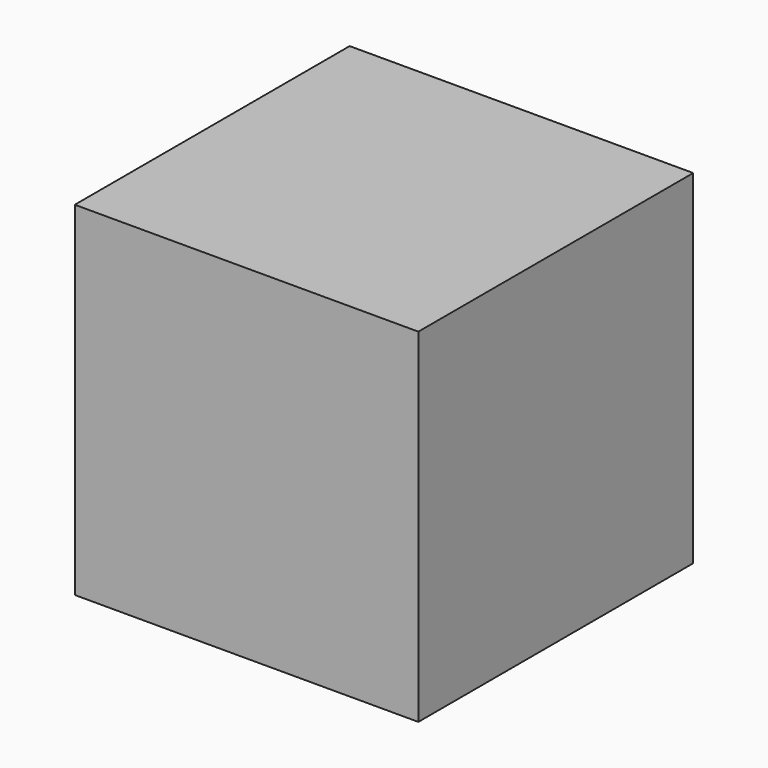
from build123d import *

# Parameters (mm, degrees)
F0_W     = 57
F0_H     = 57
F1_DEPTH = 28.5


# Not quite as in the source:
# - the program builds the solid bodies; features that only make, move or delete a surface that nothing else refers to are left out


with BuildPart() as f1:
    # F0 (on Top) → F1 (new body, symmetric)
    with BuildSketch(Plane.XY):
        Rectangle(F0_W, F0_H)
    extrude(amount=F1_DEPTH, both=True)


solid = f1.part
